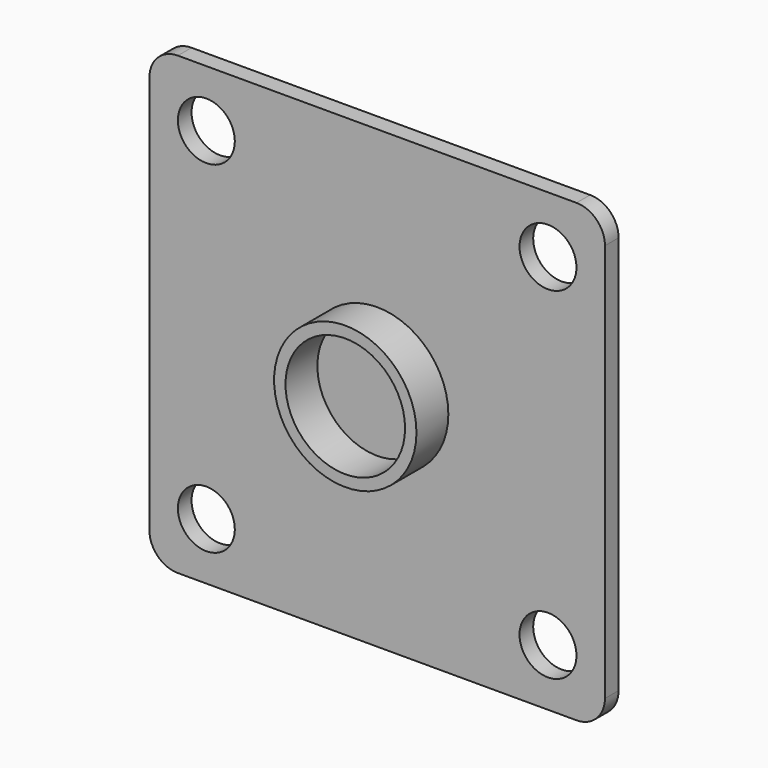
from build123d import *

# Parameters (mm, degrees)
F1_DEPTH        = 3.81
F2_R            = 6.35
F3_DEPTH        = 146
F3_DEPTH_BACK   = 25.4
F3_COPIES_COUNT = 4
F4_R            = 15.875
F4_R_2          = 13.335
F5_DEPTH        = 12.7


# Not quite as in the source:
# - an extrude ends at something that could not be found from the text; its depth is read off the source's solid
# - a pattern or mirror of a feature is missing from the dataset's text; its kind, count and spacing are read off the source's solid


with BuildPart() as f1:
    # F0 (on Front) → F1 (new body)
    with BuildSketch(Plane.XZ):
        with BuildLine():
            Line((44.45, 50.8), (-44.45, 50.8))
            ThreePointArc((-44.45, 50.8), (-48.9401280605, 48.9401280605), (-50.8, 44.45))
            Line((-50.8, 44.45), (-50.8, -44.45))
            ThreePointArc((-50.8, -44.45), (-48.9401280605, -48.9401280605), (-44.45, -50.8))
            Line((-44.45, -50.8), (44.45, -50.8))
            ThreePointArc((44.45, -50.8), (48.9401280605, -48.9401280605), (50.8, -44.45))
            Line((50.8, -44.45), (50.8, 44.45))
            ThreePointArc((50.8, 44.45), (48.9401280605, 48.9401280605), (44.45, 50.8))
        make_face()
    extrude(amount=F1_DEPTH)

    # F2 (on Front) → F3 (cut, two sides)
    with BuildSketch(Plane.XZ) as f3_sk:
        with Locations((-38.1, 38.1)):
            Circle(F2_R)
    f3 = extrude(amount=-F3_DEPTH, mode=Mode.SUBTRACT) + extrude(f3_sk.sketch, amount=F3_DEPTH_BACK, mode=Mode.SUBTRACT)

    # F3_copies: F3 ×4 about axis
    f3_copies_axis = Axis((0, 0, 0), (0, 1, 0))
    for i in range(1, F3_COPIES_COUNT):
        add(f3.rotate(f3_copies_axis, i * 360 / F3_COPIES_COUNT), mode=Mode.SUBTRACT)

    # F4 (on Front) → F5 (join)
    with BuildSketch(Plane.XZ):
        Circle(F4_R)
        Circle(F4_R_2, mode=Mode.SUBTRACT)
    extrude(amount=F5_DEPTH)


solid = f1.part
